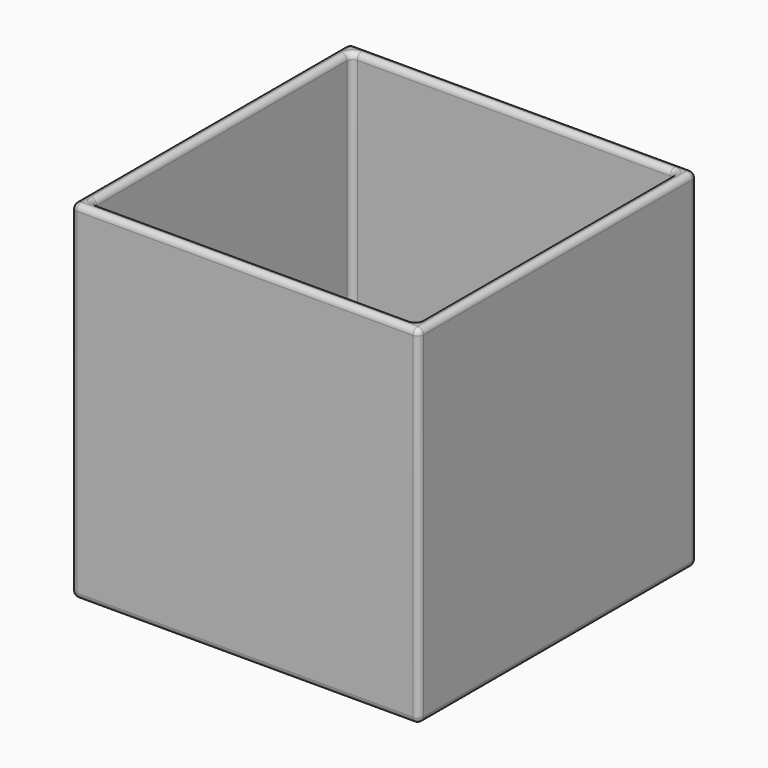
from build123d import *

# Parameters (mm, degrees)
F0_W     = 152.4
F0_H     = 152.4
F1_DEPTH = 152.4
F2_T     = -5.08
F3_R     = 2.53999


# Not quite as in the source:
# - a fillet or chamfer is up to 0.001 mm smaller than in the source, because OpenCascade refuses the exact size


with BuildPart() as f1:
    # F0 (on Top) → F1 (new body)
    with BuildSketch(Plane.XY):
        Rectangle(F0_W, F0_H)
    extrude(amount=F1_DEPTH)

    # F2
    f2_openings = [f1.faces().sort_by_distance(p)[0] for p in [
        (0, 0, 152.4),
    ]]
    offset(amount=F2_T, openings=f2_openings)

    # F3 (radius 2.54 in the source; OpenCascade refuses exactly that, so slightly less here)
    f3_edges = [f1.edges().sort_by_distance(p)[0] for p in [
        (76.2, 0, 152.4),
        (0, 76.2, 152.4),
        (-76.2, 0, 152.4),
        (0, -76.2, 152.4),
        (71.12, 0, 152.4),
        (0, -71.12, 152.4),
        (-71.12, 0, 152.4),
        (0, 71.12, 152.4),
        (76.2, 76.2, 76.2),
        (-76.2, 76.2, 76.2),
        (0, 76.2, 0),
        (71.12, 0, 5.08),
        (0, 71.12, 5.08),
        (-71.12, 0, 5.08),
        (0, -71.12, 5.08),
        (-71.12, -71.12, 78.74),
        (-71.12, 71.12, 78.74),
        (71.12, -71.12, 78.74),
        (71.12, 71.12, 78.74),
        (-76.2, -76.2, 76.2),
        (-76.2, 0, 0),
        (76.2, -76.2, 76.2),
        (0, -76.2, 0),
        (76.2, 0, 0),
    ]]
    fillet(f3_edges, radius=F3_R)


solid = f1.part
